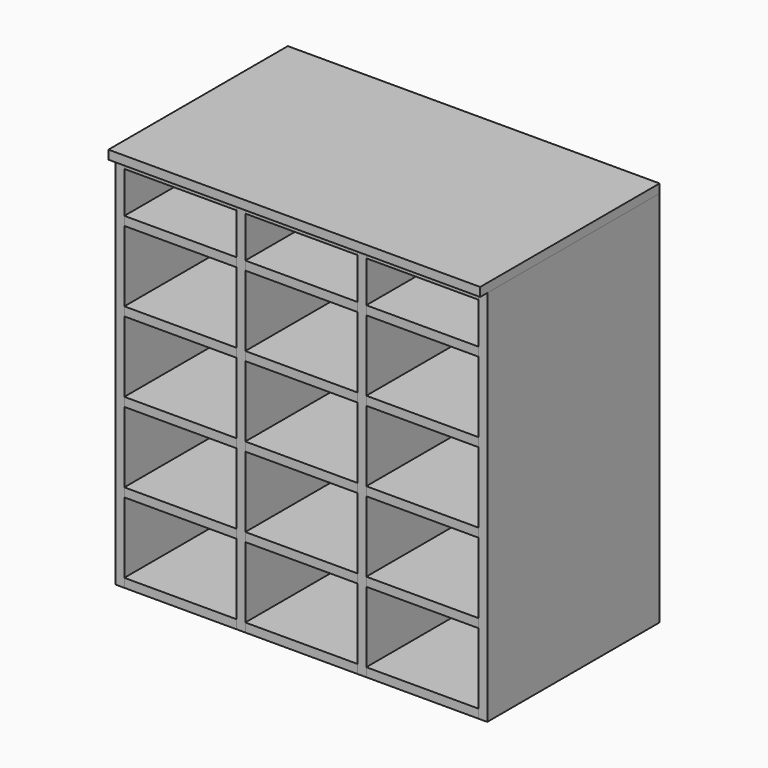
from build123d import *

# Parameters (mm, degrees)
F1_W      = 800.1
F1_H      = 482.6
F2_DEPTH  = 19.05
F3_W      = 19.05
F3_H      = 463.55
F4_DEPTH  = 812.8
F5_W      = 762
F5_H      = 19.05
F6_DEPTH  = 812.8
F7_W      = 19.05
F7_H      = 444.5
F8_DEPTH  = 812.8
F9_W      = 241.3
F9_H      = 19.05
F10_DEPTH = 444.5


# Not quite as in the source:
# - a variable given as a bare number and used for a length is read in inches; the dataset says mm whatever the document's units were


with BuildPart() as f2:
    # F1 (on Top) → F2 (new body)
    with BuildSketch(Plane.XY):
        Rectangle(F1_W, F1_H)
    extrude(amount=F2_DEPTH)


with BuildPart() as f4:
    # F3 (on face) → F4 (new body)
    with BuildSketch(Plane.XY):
        with Locations((-390.525, 9.525)):
            Rectangle(F3_W, F3_H)
    extrude(amount=-F4_DEPTH)


with BuildPart() as f4b:
    # F3 (on face) → F4, piece 2 (new body)
    with BuildSketch(Plane.XY):
        with Locations((390.525, 9.525)):
            Rectangle(F3_W, F3_H)
    extrude(amount=-F4_DEPTH)


with BuildPart() as f6:
    # F5 (on face) → F6 (new body)
    with BuildSketch(Plane.XY):
        with Locations((0, 231.775)):
            Rectangle(F5_W, F5_H)
    extrude(amount=-F6_DEPTH)


with BuildPart() as f8:
    # F7 (on face) → F8 (new body)
    with BuildSketch(Plane.XY):
        with Locations((-130.175, 0)):
            Rectangle(F7_W, F7_H)
    extrude(amount=-F8_DEPTH)


with BuildPart() as f8b:
    # F7 (on face) → F8, piece 2 (new body)
    with BuildSketch(Plane.XY):
        with Locations((130.175, 0)):
            Rectangle(F7_W, F7_H)
    extrude(amount=-F8_DEPTH)


with BuildPart() as f10:
    # F9 (on face) → F10 (new body, through all)
    with BuildSketch(Plane.XZ.offset(-222.25)):
        with Locations((-260.35, -9.525)):
            Rectangle(F9_W, F9_H)
    extrude(amount=F10_DEPTH)


with BuildPart() as f10b:
    # F9 (on face) → F10, piece 2 (new body, through all)
    with BuildSketch(Plane.XZ.offset(-222.25)):
        with Locations((260.35, -9.525)):
            Rectangle(F9_W, F9_H)
    extrude(amount=F10_DEPTH)


with BuildPart() as f10c:
    # F9 (on face) → F10, piece 3 (new body, through all)
    with BuildSketch(Plane.XZ.offset(-222.25)):
        with Locations((0, -9.525)):
            Rectangle(F9_W, F9_H)
    extrude(amount=F10_DEPTH)


with BuildPart() as f10d:
    # F9 (on face) → F10, piece 4 (new body, through all)
    with BuildSketch(Plane.XZ.offset(-222.25)):
        with Locations((-260.35, -803.275)):
            Rectangle(F9_W, F9_H)
    extrude(amount=F10_DEPTH)


with BuildPart() as f10e:
    # F9 (on face) → F10, piece 5 (new body, through all)
    with BuildSketch(Plane.XZ.offset(-222.25)):
        with Locations((260.35, -803.275)):
            Rectangle(F9_W, F9_H)
    extrude(amount=F10_DEPTH)


with BuildPart() as f10f:
    # F9 (on face) → F10, piece 6 (new body, through all)
    with BuildSketch(Plane.XZ.offset(-222.25)):
        with Locations((0, -803.275)):
            Rectangle(F9_W, F9_H)
    extrude(amount=F10_DEPTH)


with BuildPart() as f10g:
    # F9 (on face) → F10, piece 7 (new body, through all)
    with BuildSketch(Plane.XZ.offset(-222.25)):
        with Locations((260.35, -631.825)):
            Rectangle(F9_W, F9_H)
    extrude(amount=F10_DEPTH)


with BuildPart() as f10h:
    # F9 (on face) → F10, piece 8 (new body, through all)
    with BuildSketch(Plane.XZ.offset(-222.25)):
        with Locations((-260.35, -631.825)):
            Rectangle(F9_W, F9_H)
    extrude(amount=F10_DEPTH)


with BuildPart() as f10i:
    # F9 (on face) → F10, piece 9 (new body, through all)
    with BuildSketch(Plane.XZ.offset(-222.25)):
        with Locations((0, -631.825)):
            Rectangle(F9_W, F9_H)
    extrude(amount=F10_DEPTH)


with BuildPart() as f10j:
    # F9 (on face) → F10, piece 10 (new body, through all)
    with BuildSketch(Plane.XZ.offset(-222.25)):
        with Locations((260.35, -460.375)):
            Rectangle(F9_W, F9_H)
    extrude(amount=F10_DEPTH)


with BuildPart() as f10k:
    # F9 (on face) → F10, piece 11 (new body, through all)
    with BuildSketch(Plane.XZ.offset(-222.25)):
        with Locations((-260.35, -460.375)):
            Rectangle(F9_W, F9_H)
    extrude(amount=F10_DEPTH)


with BuildPart() as f10l:
    # F9 (on face) → F10, piece 12 (new body, through all)
    with BuildSketch(Plane.XZ.offset(-222.25)):
        with Locations((0, -460.375)):
            Rectangle(F9_W, F9_H)
    extrude(amount=F10_DEPTH)


with BuildPart() as f10m:
    # F9 (on face) → F10, piece 13 (new body, through all)
    with BuildSketch(Plane.XZ.offset(-222.25)):
        with Locations((260.35, -288.925)):
            Rectangle(F9_W, F9_H)
    extrude(amount=F10_DEPTH)


with BuildPart() as f10n:
    # F9 (on face) → F10, piece 14 (new body, through all)
    with BuildSketch(Plane.XZ.offset(-222.25)):
        with Locations((-260.35, -288.925)):
            Rectangle(F9_W, F9_H)
    extrude(amount=F10_DEPTH)


with BuildPart() as f10o:
    # F9 (on face) → F10, piece 15 (new body, through all)
    with BuildSketch(Plane.XZ.offset(-222.25)):
        with Locations((0, -288.925)):
            Rectangle(F9_W, F9_H)
    extrude(amount=F10_DEPTH)


with BuildPart() as f10p:
    # F9 (on face) → F10, piece 16 (new body, through all)
    with BuildSketch(Plane.XZ.offset(-222.25)):
        with Locations((260.35, -117.475)):
            Rectangle(F9_W, F9_H)
    extrude(amount=F10_DEPTH)


with BuildPart() as f10q:
    # F9 (on face) → F10, piece 17 (new body, through all)
    with BuildSketch(Plane.XZ.offset(-222.25)):
        with Locations((-260.35, -117.475)):
            Rectangle(F9_W, F9_H)
    extrude(amount=F10_DEPTH)


with BuildPart() as f10r:
    # F9 (on face) → F10, piece 18 (new body, through all)
    with BuildSketch(Plane.XZ.offset(-222.25)):
        with Locations((0, -117.475)):
            Rectangle(F9_W, F9_H)
    extrude(amount=F10_DEPTH)


solid = Compound([f2.part, f4.part, f4b.part, f6.part, f8.part, f8b.part, f10.part, f10b.part, f10c.part, f10d.part, f10e.part, f10f.part, f10g.part, f10h.part, f10i.part, f10j.part, f10k.part, f10l.part, f10m.part, f10n.part, f10o.part, f10p.part, f10q.part, f10r.part])
